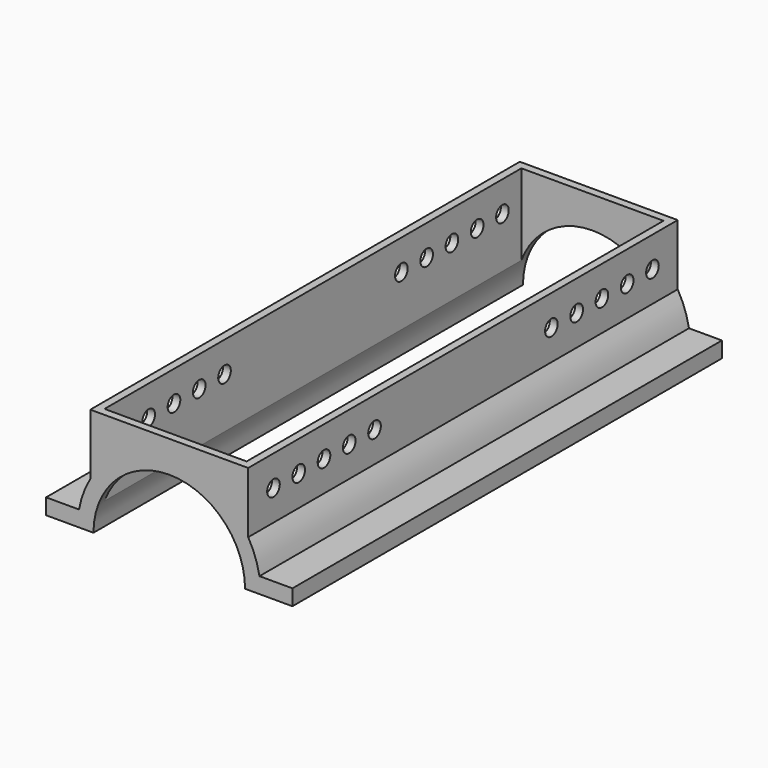
from build123d import *

# Parameters (mm, degrees)
F1_DEPTH = 215.9
F2_W     = 57.15
F2_H     = 209.55
F3_DEPTH = 32.5744088888
F4_R     = 3.175
F5_DEPTH = 81.281


# Not quite as in the source:
# - a feature names something its author has since deleted; it is built from what else it names


with BuildPart() as f1:
    # F0 (on Front) → F1 (new body)
    with BuildSketch(Plane.XZ):
        with BuildLine():
            Line((-36.83, 0), (-30.48, 0))
            ThreePointArc((-30.48, 0), (0, 30.48), (30.48, 0))
            Line((30.48, 0), (36.83, 0))
            Line((36.83, 0), (49.53, 0))
            Line((49.53, 0), (49.53, 6.35))
            Line((49.53, 6.35), (36.278456417, 6.35))
            ThreePointArc((36.278456417, 6.35), (34.5670828322, 12.7108490854), (31.75, 18.66511184))
            ThreePointArc((31.75, 18.66511184), (30.2489666674, 21.0106857469), (28.575, 23.2361415687))
            ThreePointArc((28.575, 23.2361415687), (0, 36.83), (-28.575, 23.2361415687))
            ThreePointArc((-28.575, 23.2361415687), (-30.2489666674, 21.0106857469), (-31.75, 18.66511184))
            ThreePointArc((-31.75, 18.66511184), (-34.5670828322, 12.7108490854), (-36.278456417, 6.35))
            Line((-36.278456417, 6.35), (-49.53, 6.35))
            Line((-49.53, 6.35), (-49.53, 0))
            Line((-49.53, 0), (-36.83, 0))
        make_face()
        with BuildLine():
            ThreePointArc((28.575, 23.2361415687), (30.2489666674, 21.0106857469), (31.75, 18.66511184))
            Line((31.75, 18.66511184), (31.75, 43.18))
            Line((31.75, 43.18), (28.575, 43.18))
            Line((28.575, 43.18), (28.575, 23.2361415687))
        make_face()
        with BuildLine():
            Line((-28.575, 43.18), (-28.575, 23.2361415687))
            ThreePointArc((-28.575, 23.2361415687), (0, 36.83), (28.575, 23.2361415687))
            Line((28.575, 23.2361415687), (28.575, 43.18))
            Line((28.575, 43.18), (-28.575, 43.18))
        make_face()
        with BuildLine():
            Line((-31.75, 43.18), (-31.75, 18.66511184))
            ThreePointArc((-31.75, 18.66511184), (-30.2489666674, 21.0106857469), (-28.575, 23.2361415687))
            Line((-28.575, 23.2361415687), (-28.575, 43.18))
            Line((-28.575, 43.18), (-31.75, 43.18))
        make_face()
    extrude(amount=-F1_DEPTH)

    # F2 (on face) → F3 (cut, through all)
    with BuildSketch(Plane.XY.offset(43.18)):
        with Locations((0, 107.95)):
            Rectangle(F2_W, F2_H)
    extrude(amount=-F3_DEPTH, mode=Mode.SUBTRACT)

    # F4 (on face) → F5 (cut, through all)
    with BuildSketch(Plane.YZ.offset(31.75)):
        with Locations((12.7, 30.92255592)):
            Circle(F4_R)
        with Locations((25.4, 30.92255592)):
            Circle(F4_R)
        with Locations((38.1, 30.92255592)):
            Circle(F4_R)
        with Locations((50.8, 30.92255592)):
            Circle(F4_R)
        with Locations((63.5, 30.92255592)):
            Circle(F4_R)
        with Locations((152.4, 30.92255592)):
            Circle(F4_R)
        with Locations((165.1, 30.92255592)):
            Circle(F4_R)
        with Locations((177.8, 30.92255592)):
            Circle(F4_R)
        with Locations((190.5, 30.92255592)):
            Circle(F4_R)
        with Locations((203.2, 30.92255592)):
            Circle(F4_R)
    extrude(amount=-F5_DEPTH, mode=Mode.SUBTRACT)


solid = f1.part
